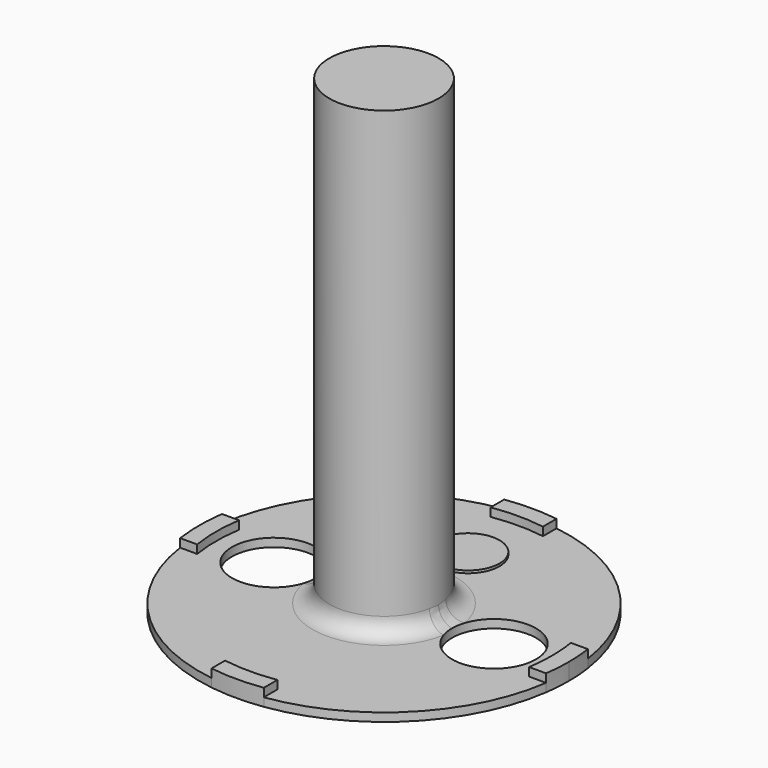
from build123d import *

# Parameters (mm, degrees)
F0_R     = 12.7
F0_R_2   = 16.51
F1_DEPTH = 2.54
F2_DEPTH = 5.08
F3_DEPTH = 142.24
F4_R     = 5.08
F6_DEPTH = 0.762


with BuildPart() as f1:
    # F0 (on Top) → F1 (new body)
    with BuildSketch(Plane.XY):
        with BuildLine():
            ThreePointArc((55.317317, -7.910045), (55.739152, -3.965017), (55.88, 0))
            ThreePointArc((55.88, 0), (55.739152, 3.965017), (55.317317, 7.910045))
            Line((55.317317, 7.910045), (50.180386, 7.910045))
            ThreePointArc((50.180386, 7.910045), (50.64486, 3.967138), (50.8, 0))
            ThreePointArc((50.8, 0), (50.64486, -3.967138), (50.180386, -7.910045))
            Line((50.180386, -7.910045), (55.317317, -7.910045))
        make_face()
        with BuildLine():
            Line((50.180386, 7.910045), (55.317317, 7.910045))
            ThreePointArc((55.317317, 7.910045), (39.513127, 39.513127), (7.910045, 55.317317))
            Line((7.910045, 55.317317), (7.910045, 50.180386))
            ThreePointArc((7.910045, 50.180386), (35.921024, 35.921024), (50.180386, 7.910045))
        make_face()
        with BuildLine():
            ThreePointArc((7.910045, -55.317317), (39.513127, -39.513127), (55.317317, -7.910045))
            Line((55.317317, -7.910045), (50.180386, -7.910045))
            ThreePointArc((50.180386, -7.910045), (35.921024, -35.921024), (7.910045, -50.180386))
            Line((7.910045, -50.180386), (7.910045, -55.317317))
        make_face()
        with BuildLine():
            Line((7.910045, 50.180386), (7.910045, 55.317317))
            ThreePointArc((7.910045, 55.317317), (0, 55.88), (-7.910045, 55.317317))
            Line((-7.910045, 55.317317), (-7.910045, 50.180386))
            ThreePointArc((-7.910045, 50.180386), (0, 50.8), (7.910045, 50.180386))
        make_face()
        with BuildLine():
            ThreePointArc((-7.910045, -55.317317), (0, -55.88), (7.910045, -55.317317))
            Line((7.910045, -55.317317), (7.910045, -50.180386))
            ThreePointArc((7.910045, -50.180386), (0, -50.8), (-7.910045, -50.180386))
            Line((-7.910045, -50.180386), (-7.910045, -55.317317))
        make_face()
        with BuildLine():
            Line((-7.910045, 50.180386), (-7.910045, 55.317317))
            ThreePointArc((-7.910045, 55.317317), (-39.513127, 39.513127), (-55.317317, 7.910045))
            Line((-55.317317, 7.910045), (-50.180386, 7.910045))
            ThreePointArc((-50.180386, 7.910045), (-35.921024, 35.921024), (-7.910045, 50.180386))
        make_face()
        with BuildLine():
            ThreePointArc((-55.317317, -7.910045), (-39.513127, -39.513127), (-7.910045, -55.317317))
            Line((-7.910045, -55.317317), (-7.910045, -50.180386))
            ThreePointArc((-7.910045, -50.180386), (-35.921024, -35.921024), (-50.180386, -7.910045))
            Line((-50.180386, -7.910045), (-55.317317, -7.910045))
        make_face()
        with BuildLine():
            Line((-50.180386, 7.910045), (-55.317317, 7.910045))
            ThreePointArc((-55.317317, 7.910045), (-55.88, 0), (-55.317317, -7.910045))
            Line((-55.317317, -7.910045), (-50.180386, -7.910045))
            ThreePointArc((-50.180386, -7.910045), (-50.8, 0), (-50.180386, 7.910045))
        make_face()
        with BuildLine():
            ThreePointArc((50.8, 0), (50.64486, 3.967138), (50.180386, 7.910045))
            ThreePointArc((50.180386, 7.910045), (35.921024, 35.921024), (7.910045, 50.180386))
            ThreePointArc((7.910045, 50.180386), (0, 50.8), (-7.910045, 50.180386))
            ThreePointArc((-7.910045, 50.180386), (-35.921024, 35.921024), (-50.180386, 7.910045))
            ThreePointArc((-50.180386, 7.910045), (-50.8, 0), (-50.180386, -7.910045))
            ThreePointArc((-50.180386, -7.910045), (-35.921024, -35.921024), (-7.910045, -50.180386))
            ThreePointArc((-7.910045, -50.180386), (0, -50.8), (7.910045, -50.180386))
            ThreePointArc((7.910045, -50.180386), (35.921024, -35.921024), (50.180386, -7.910045))
            ThreePointArc((50.180386, -7.910045), (50.64486, -3.967138), (50.8, 0))
        make_face()
        with Locations((-33.261735, 0)):
            Circle(F0_R, mode=Mode.SUBTRACT)
        Circle(F0_R_2, mode=Mode.SUBTRACT)
        with Locations((33.261735, 0)):
            Circle(F0_R, mode=Mode.SUBTRACT)
        Circle(F0_R_2)
    extrude(amount=F1_DEPTH)

    # F0 (on Top) → F2 (join)
    with BuildSketch(Plane.XY):
        with BuildLine():
            Line((-50.180386, 7.910045), (-55.317317, 7.910045))
            ThreePointArc((-55.317317, 7.910045), (-55.88, 0), (-55.317317, -7.910045))
            Line((-55.317317, -7.910045), (-50.180386, -7.910045))
            ThreePointArc((-50.180386, -7.910045), (-50.8, 0), (-50.180386, 7.910045))
        make_face()
        with BuildLine():
            Line((7.910045, 50.180386), (7.910045, 55.317317))
            ThreePointArc((7.910045, 55.317317), (0, 55.88), (-7.910045, 55.317317))
            Line((-7.910045, 55.317317), (-7.910045, 50.180386))
            ThreePointArc((-7.910045, 50.180386), (0, 50.8), (7.910045, 50.180386))
        make_face()
        with BuildLine():
            ThreePointArc((55.317317, -7.910045), (55.739152, -3.965017), (55.88, 0))
            ThreePointArc((55.88, 0), (55.739152, 3.965017), (55.317317, 7.910045))
            Line((55.317317, 7.910045), (50.180386, 7.910045))
            ThreePointArc((50.180386, 7.910045), (50.64486, 3.967138), (50.8, 0))
            ThreePointArc((50.8, 0), (50.64486, -3.967138), (50.180386, -7.910045))
            Line((50.180386, -7.910045), (55.317317, -7.910045))
        make_face()
        with BuildLine():
            ThreePointArc((-7.910045, -55.317317), (0, -55.88), (7.910045, -55.317317))
            Line((7.910045, -55.317317), (7.910045, -50.180386))
            ThreePointArc((7.910045, -50.180386), (0, -50.8), (-7.910045, -50.180386))
            Line((-7.910045, -50.180386), (-7.910045, -55.317317))
        make_face()
    extrude(amount=F2_DEPTH)

    # F0 (on Top) → F3 (join)
    with BuildSketch(Plane.XY):
        Circle(F0_R_2)
    extrude(amount=F3_DEPTH)

    # F4
    f4_edges = [f1.edges().sort_by_distance(p)[0] for p in [
        (-16.51, 0, 2.54),
    ]]
    fillet(f4_edges, radius=F4_R)

    # F5 (on face) → F6 (join)
    with BuildSketch(Plane.XY.offset(2.54)):
        with BuildLine():
            ThreePointArc((0, 22.225), (6.735192, 25.014808), (9.525, 31.75))
            ThreePointArc((9.525, 31.75), (-6.735192, 38.485192), (0, 22.225))
        make_face()
    extrude(amount=F6_DEPTH)


solid = f1.part
